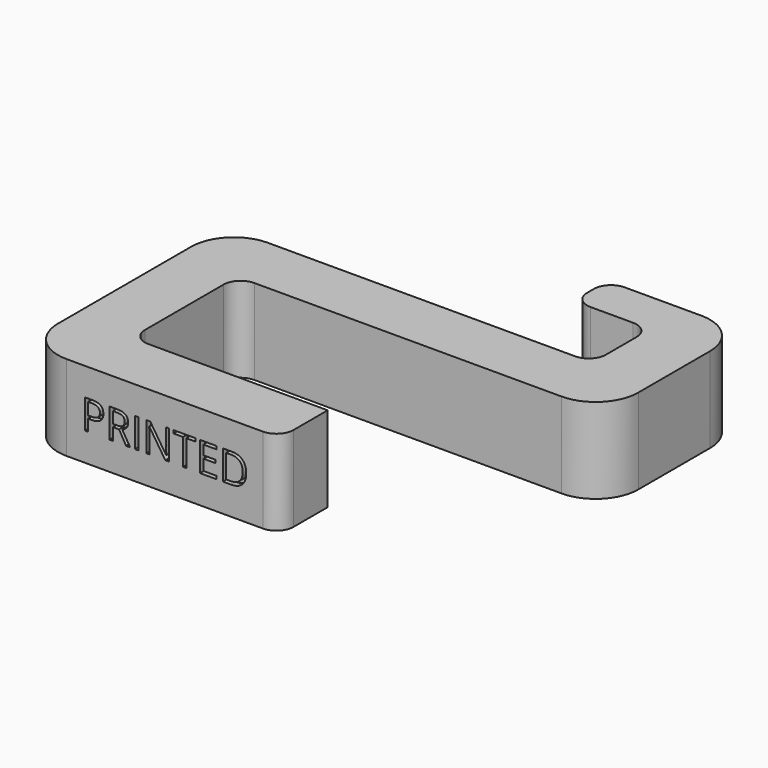
from build123d import *

# Parameters (mm, degrees)
F0_W         = 7
F0_H         = 8.5
F0_H_2       = 15.5
F1_DEPTH     = 10
F2_R         = 5
F3_R         = 2
F4_TEXT_SIZE = 4.8102189088
F5_DEPTH     = 0.7


# Not quite as in the source:
# - Text() gives the source's letters only with a copy of the font that has no kerning and outlines rounded to 1/6400 em; it was checked with that copy


with BuildPart() as f1:
    # F0 (on Top) → F1 (new body)
    with BuildSketch(Plane.XY):
        Polygon((13, 7), (-30, 7), (-30, 0), (-23, 0), (20, 0), (20, 7), align=None)
        with Locations((16.5, 11.25)):
            Rectangle(F0_W, F0_H)
        with Locations((-26.5, -7.75)):
            Rectangle(F0_W, F0_H_2)
        Polygon((4, 15.5), (13, 15.5), (20, 15.5), (20, 20.5), (4, 20.5), align=None)
        Polygon((-23, -15.5), (-30, -15.5), (-30, -22.5), (0, -22.5), (0, -15.5), align=None)
    extrude(amount=F1_DEPTH)

    # F2
    f2_edges = [f1.edges().sort_by_distance(p)[0] for p in [
        (-30, -22.5, 5),
        (-30, 7, 5),
        (20, 0, 5),
        (20, 20.5, 5),
    ]]
    fillet(f2_edges, radius=F2_R)

    # F3
    f3_edges = [f1.edges().sort_by_distance(p)[0] for p in [
        (-23, 0, 5),
        (-23, -15.5, 5),
        (0, -22.5, 5),
        (4, 20.5, 5),
        (4, 15.5, 5),
        (13, 15.5, 5),
        (13, 7, 5),
    ]]
    fillet(f3_edges, radius=F3_R)

    # F4 (on face) → F5 (cut)
    with BuildSketch(Plane.XZ.offset(22.5)):
        with Locations((-23.3288538472, 3.3180452236)):
            Text('PRINTED', F4_TEXT_SIZE, font='Open Sans', text_align=(TextAlign.LEFT, TextAlign.BOTTOM))
    extrude(amount=-F5_DEPTH, mode=Mode.SUBTRACT)


solid = f1.part
